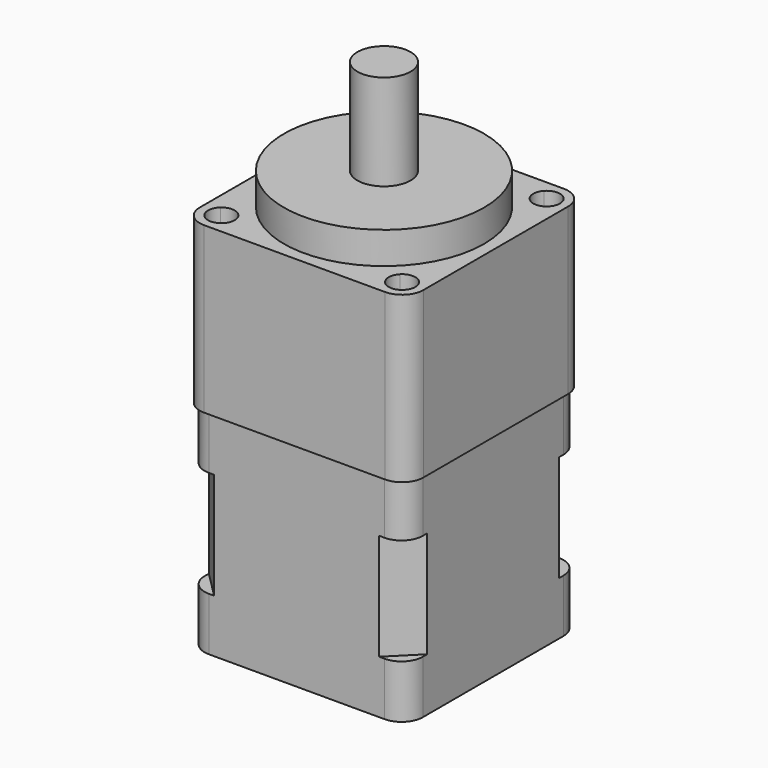
from build123d import *

# Parameters (mm, degrees)
F1_DEPTH     = 31
F2_R         = 18.8
F3_DEPTH     = 6
F4_R         = 5
F5_DEPTH     = 18
F6_R         = 4
F8_W         = 41
F8_H         = 41
F9_DEPTH     = 10
F10_T1_DEPTH = 20
F12_DEPTH    = 20
F13_W        = 41
F13_H        = 41
F14_DEPTH    = 10
F15_R        = 4


# Not quite as in the source:
# - a fillet or chamfer that OpenCascade refuses, or shapes differently, is made with other operations: its cross-section is extruded or revolved along the edge and cut away or added


with BuildPart() as f1:
    # F0 (on Top) → F1 (new body)
    with BuildSketch(Plane.XY):
        with BuildLine():
            Line((18.7383297014, 18.7383297014), (21, 21))
            Line((21, 21), (11.6189500386, 21))
            ThreePointArc((11.6189500386, 21), (13.4178535673, 19.8987739735), (15.1131239157, 18.6438591903))
            ThreePointArc((15.1131239157, 18.6438591903), (16.9054364798, 19.4697143183), (18.7383297014, 18.7383297014))
        make_face()
        with BuildLine():
            ThreePointArc((-15.1131239157, 18.6438591903), (-13.4178535673, 19.8987739735), (-11.6189500386, 21))
            Line((-11.6189500386, 21), (-21, 21))
            Line((-21, 21), (-18.7383297014, 18.7383297014))
            ThreePointArc((-18.7383297014, 18.7383297014), (-16.9054364798, 19.4697143183), (-15.1131239157, 18.6438591903))
        make_face()
        with BuildLine():
            Line((11.6189500386, -21), (21, -21))
            Line((21, -21), (18.7383297014, -18.7383297014))
            ThreePointArc((18.7383297014, -18.7383297014), (16.9054364798, -19.4697143183), (15.1131239157, -18.6438591903))
            ThreePointArc((15.1131239157, -18.6438591903), (13.4178535673, -19.8987739735), (11.6189500386, -21))
        make_face()
        with BuildLine():
            Line((-21, -21), (-11.6189500386, -21))
            ThreePointArc((-11.6189500386, -21), (-13.4178535673, -19.8987739735), (-15.1131239157, -18.6438591903))
            ThreePointArc((-15.1131239157, -18.6438591903), (-16.9054364798, -19.4697143183), (-18.7383297014, -18.7383297014))
            Line((-18.7383297014, -18.7383297014), (-21, -21))
        make_face()
        with BuildLine():
            Line((21, 11.6189500386), (21, 21))
            Line((21, 21), (18.7383297014, 18.7383297014))
            ThreePointArc((18.7383297014, 18.7383297014), (19.2802615798, 17.9272713294), (19.4705627485, 16.9705627485))
            ThreePointArc((19.4705627485, 16.9705627485), (19.2545549885, 15.954010021), (18.6438591903, 15.1131239157))
            ThreePointArc((18.6438591903, 15.1131239157), (19.8987739735, 13.4178535673), (21, 11.6189500386))
        make_face()
        with BuildLine():
            Line((21, -21), (21, -11.6189500386))
            ThreePointArc((21, -11.6189500386), (19.8987739735, -13.4178535673), (18.6438591903, -15.1131239157))
            ThreePointArc((18.6438591903, -15.1131239157), (19.2545549885, -15.954010021), (19.4705627485, -16.9705627485))
            ThreePointArc((19.4705627485, -16.9705627485), (19.2802615798, -17.9272713294), (18.7383297014, -18.7383297014))
            Line((18.7383297014, -18.7383297014), (21, -21))
        make_face()
        with BuildLine():
            Line((-18.7383297014, 18.7383297014), (-21, 21))
            Line((-21, 21), (-21, 11.6189500386))
            ThreePointArc((-21, 11.6189500386), (-19.8987739735, 13.4178535673), (-18.6438591903, 15.1131239157))
            ThreePointArc((-18.6438591903, 15.1131239157), (-19.4697143183, 16.9054364798), (-18.7383297014, 18.7383297014))
        make_face()
        with BuildLine():
            ThreePointArc((-18.6438591903, -15.1131239157), (-19.8987739735, -13.4178535673), (-21, -11.6189500386))
            Line((-21, -11.6189500386), (-21, -21))
            Line((-21, -21), (-18.7383297014, -18.7383297014))
            ThreePointArc((-18.7383297014, -18.7383297014), (-19.4697143183, -16.9054364798), (-18.6438591903, -15.1131239157))
        make_face()
        with BuildLine():
            ThreePointArc((15.1131239157, 18.6438591903), (13.4178535673, 19.8987739735), (11.6189500386, 21))
            Line((11.6189500386, 21), (-11.6189500386, 21))
            ThreePointArc((-11.6189500386, 21), (-13.4178535673, 19.8987739735), (-15.1131239157, 18.6438591903))
            ThreePointArc((-15.1131239157, 18.6438591903), (-14.6367250204, 17.8667778225), (-14.4705627485, 16.9705627485))
            ThreePointArc((-14.4705627485, 16.9705627485), (-14.6608639172, 16.0138541676), (-15.2027957955, 15.2027957955))
            Line((-15.2027957955, 15.2027957955), (0, 0))
            Line((0, 0), (15.2027957955, 15.2027957955))
            ThreePointArc((15.2027957955, 15.2027957955), (14.4714111786, 16.9054364798), (15.1131239157, 18.6438591903))
        make_face()
        with BuildLine():
            Line((15.2027957955, -15.2027957955), (0, 0))
            Line((0, 0), (-15.2027957955, -15.2027957955))
            ThreePointArc((-15.2027957955, -15.2027957955), (-14.6608639172, -16.0138541676), (-14.4705627485, -16.9705627485))
            ThreePointArc((-14.4705627485, -16.9705627485), (-14.6367250204, -17.8667778225), (-15.1131239157, -18.6438591903))
            ThreePointArc((-15.1131239157, -18.6438591903), (-13.4178535673, -19.8987739735), (-11.6189500386, -21))
            Line((-11.6189500386, -21), (11.6189500386, -21))
            ThreePointArc((11.6189500386, -21), (13.4178535673, -19.8987739735), (15.1131239157, -18.6438591903))
            ThreePointArc((15.1131239157, -18.6438591903), (14.4714111786, -16.9054364798), (15.2027957955, -15.2027957955))
        make_face()
        with BuildLine():
            Line((21, -11.6189500386), (21, 11.6189500386))
            ThreePointArc((21, 11.6189500386), (19.8987739735, 13.4178535673), (18.6438591903, 15.1131239157))
            ThreePointArc((18.6438591903, 15.1131239157), (16.9054364798, 14.4714111786), (15.2027957955, 15.2027957955))
            Line((15.2027957955, 15.2027957955), (0, 0))
            Line((0, 0), (15.2027957955, -15.2027957955))
            ThreePointArc((15.2027957955, -15.2027957955), (16.9054364798, -14.4714111786), (18.6438591903, -15.1131239157))
            ThreePointArc((18.6438591903, -15.1131239157), (19.8987739735, -13.4178535673), (21, -11.6189500386))
        make_face()
        with BuildLine():
            ThreePointArc((-18.6438591903, 15.1131239157), (-19.8987739735, 13.4178535673), (-21, 11.6189500386))
            Line((-21, 11.6189500386), (-21, -11.6189500386))
            ThreePointArc((-21, -11.6189500386), (-19.8987739735, -13.4178535673), (-18.6438591903, -15.1131239157))
            ThreePointArc((-18.6438591903, -15.1131239157), (-16.9054364798, -14.4714111786), (-15.2027957955, -15.2027957955))
            Line((-15.2027957955, -15.2027957955), (0, 0))
            Line((0, 0), (-15.2027957955, 15.2027957955))
            ThreePointArc((-15.2027957955, 15.2027957955), (-16.9054364798, 14.4714111786), (-18.6438591903, 15.1131239157))
        make_face()
    extrude(amount=F1_DEPTH)

    # F2 (on face) → F3 (join)
    with BuildSketch(Plane.XY.offset(31)):
        Circle(F2_R)
    extrude(amount=F3_DEPTH)

    # F4 (on face) → F5 (join)
    with BuildSketch(Plane.XY.offset(37)):
        Circle(F4_R)
    extrude(amount=F5_DEPTH)

    # F6
    f6_edges = [f1.edges().sort_by_distance(p)[0] for p in [
        (-21, -21, 15.5),
        (-21, 21, 15.5),
        (21, 21, 15.5),
        (21, -21, 15.5),
    ]]
    fillet(f6_edges, radius=F6_R)

    # F8 (on face) → F9 (join)
    with BuildSketch(Plane(origin=(0, 0, 0), x_dir=(1, 0, 0), z_dir=(0, 0, -1))):
        Rectangle(F8_W, F8_H)
    extrude(amount=F9_DEPTH)

    # F10: fillet of radius 4 on 4 edges, made by hand

    # F10_s2 → F10_t1 (cut)
    with BuildSketch(Plane.XY.offset(-20)):
        with BuildLine():
            ThreePointArc((20.5, -16.5), (19.3284271247, -19.3284271247), (16.5, -20.5))
            Line((16.5, -20.5), (20.5, -20.5))
            Line((20.5, -20.5), (20.5, -16.5))
        make_face()
        with BuildLine():
            ThreePointArc((16.5, 20.5), (19.3284271247, 19.3284271247), (20.5, 16.5))
            Line((20.5, 16.5), (20.5, 20.5))
            Line((20.5, 20.5), (16.5, 20.5))
        make_face()
        with BuildLine():
            ThreePointArc((-16.5, 20.5), (-19.3284271247, 19.3284271247), (-20.5, 16.5))
            Line((-20.5, 16.5), (-20.5, 20.5))
            Line((-20.5, 20.5), (-16.5, 20.5))
        make_face()
        with BuildLine():
            ThreePointArc((-20.5, -16.5), (-19.3284271247, -19.3284271247), (-16.5, -20.5))
            Line((-16.5, -20.5), (-20.5, -20.5))
            Line((-20.5, -20.5), (-20.5, -16.5))
        make_face()
    extrude(amount=F10_T1_DEPTH, mode=Mode.SUBTRACT)

    # F11 (on face) → F12 (join)
    with BuildSketch(Plane(origin=(0, 0, -10), x_dir=(1, 0, 0), z_dir=(0, 0, -1))):
        Polygon((-15.5, 20.5), (-20.5, 15.5), (-15.5, 15.5), align=None)
        Polygon((15.5, 15.5), (20.5, 15.5), (15.5, 20.5), align=None)
        Polygon((15.5, -15.5), (15.5, -20.5), (20.5, -15.5), align=None)
        Polygon((-20.5, -15.5), (-15.5, -20.5), (-15.5, -15.5), align=None)
        Polygon((-15.5, -20.5), (15.5, -20.5), (15.5, -15.5), (20.5, -15.5), (20.5, 15.5), (15.5, 15.5), (15.5, 20.5), (-15.5, 20.5), (-15.5, 15.5), (-20.5, 15.5), (-20.5, -15.5), (-15.5, -15.5), align=None)
    extrude(amount=F12_DEPTH)

    # F13 (on face) → F14 (join)
    with BuildSketch(Plane(origin=(0, 0, -30), x_dir=(1, 0, 0), z_dir=(0, 0, -1))):
        Rectangle(F13_W, F13_H)
    extrude(amount=F14_DEPTH)

    # F15
    f15_edges = [f1.edges().sort_by_distance(p)[0] for p in [
        (20.5, -20.5, -35),
        (-20.5, -20.5, -35),
        (20.5, 20.5, -35),
        (-20.5, 20.5, -35),
    ]]
    fillet(f15_edges, radius=F15_R)


solid = f1.part
